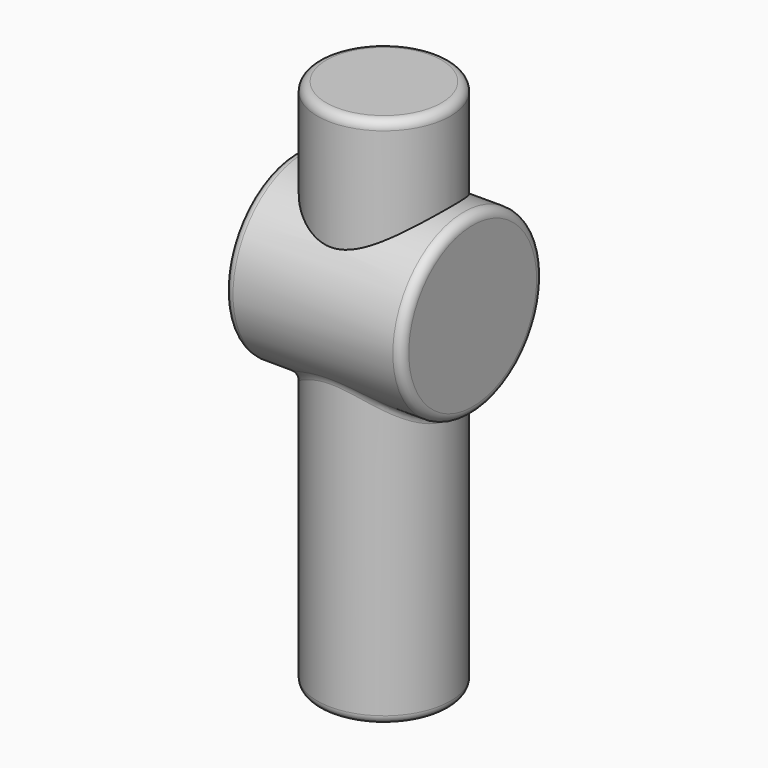
from build123d import *

# Parameters (mm, degrees)
F0_R     = 12.7
F1_DEPTH = 12.7
F2_R     = 9.525
F3_DEPTH = 25.4
F4_R     = 9.525
F5_DEPTH = 25.4
F6_R     = 1.27


with BuildPart() as f1:
    # F0 (on Right) → F1 (new body, symmetric)
    with BuildSketch(Plane.YZ):
        Circle(F0_R)
    extrude(amount=F1_DEPTH, both=True)

    # F2 (on Top) → F3 (join, symmetric)
    with BuildSketch(Plane.XY):
        Circle(F2_R)
    extrude(amount=F3_DEPTH, both=True)

    # F4 (on face) → F5 (join)
    with BuildSketch(Plane(origin=(0, 0, -25.4), x_dir=(1, 0, 0), z_dir=(0, 0, -1))):
        Circle(F4_R)
    extrude(amount=F5_DEPTH)

    # F6
    f6_edges = [f1.edges().sort_by_distance(p)[0] for p in [
        (12.7, -12.7, 0),
        (-12.7, -12.7, 0),
        (-9.525, 0, 25.4),
        (-9.525, 0, -12.7),
        (9.525, 0, -31.75),
        (-9.525, 0, -50.8),
    ]]
    fillet(f6_edges, radius=F6_R)


solid = f1.part
